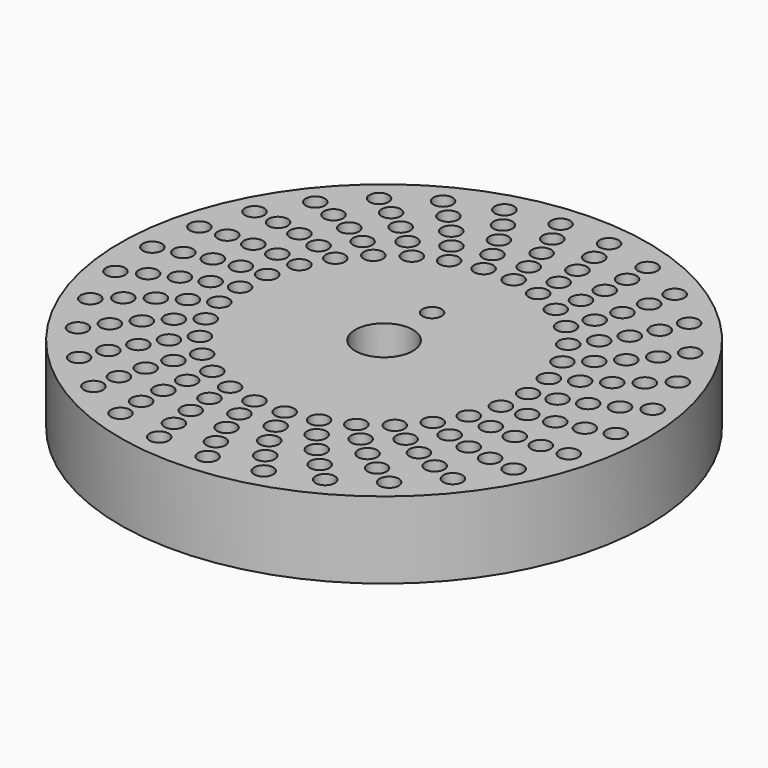
from build123d import *

# Parameters (mm, degrees)
F0_R            = 55
F0_R_2          = 6
F1_DEPTH        = 16
F3_D            = 4
F3_COPIES_COUNT = 30
F5_D            = 4


# Not quite as in the source:
# - a pattern or mirror of a feature is missing from the dataset's text; its kind, count and spacing are read off the source's solid


with BuildPart() as f1:
    # F0 (on Top) → F1 (new body)
    with BuildSketch(Plane.XY):
        Circle(F0_R)
        Circle(F0_R_2, mode=Mode.SUBTRACT)
    extrude(amount=F1_DEPTH)

    # F3 (through all)
    with Locations(Plane.XY.offset(16)):
        with Locations((30, 0), (34.9692990535, 1.4656478805), (39.85971437, 3.3471137333), (44.6451615592, 5.6399955104), (49.2998018535, 8.3384373358)):
            f3 = Hole(F3_D / 2)

    # F3_copies: F3 ×30 about axis
    f3_copies_axis = Axis((0, 0, 0), (0, 0, 1))
    for i in range(1, F3_COPIES_COUNT):
        add(f3.rotate(f3_copies_axis, i * 360 / F3_COPIES_COUNT), mode=Mode.SUBTRACT)

    # F5 (through all)
    with Locations(Plane.XY.offset(16)):
        with Locations((0, 12.5)):
            Hole(F5_D / 2)


solid = f1.part
